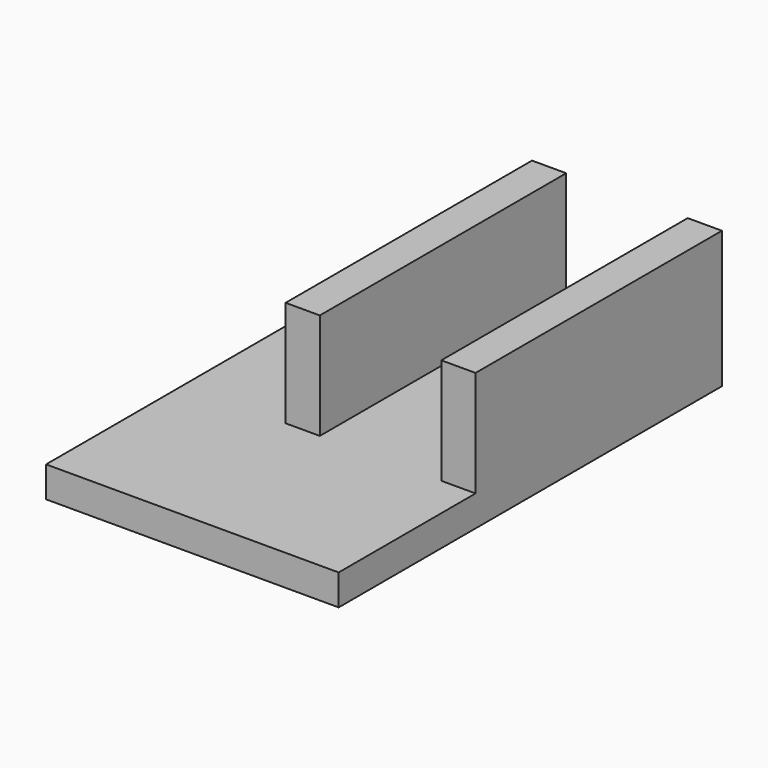
from build123d import *

# Parameters (mm, degrees)
F0_W     = 7.1
F0_H     = 18
F1_DEPTH = 1.8
F0_W_2   = 2
F2_DEPTH = 8


# Not quite as in the source:
# - a feature names something its author has since deleted; it is built from what else it names


with BuildPart() as f1:
    # F0 (on Top) → F1 (new body)
    with BuildSketch(Plane.XY):
        Polygon((5.55, -9), (3.55, -9), (-3.55, -9), (-5.55, -9), (-5.55, -19), (5.55, -19), align=None)
        Rectangle(F0_W, F0_H)
        Polygon((-5.55, -19), (-5.55, -9), (-5.55, 9), (-11.55, 9), (-11.55, -19), align=None)
    extrude(amount=F1_DEPTH)

    # F0 (on Top) → F2 (join)
    with BuildSketch(Plane.XY):
        with Locations((-4.55, 0)):
            Rectangle(F0_W_2, F0_H)
        with Locations((4.55, 0)):
            Rectangle(F0_W_2, F0_H)
    extrude(amount=F2_DEPTH)


solid = f1.part
